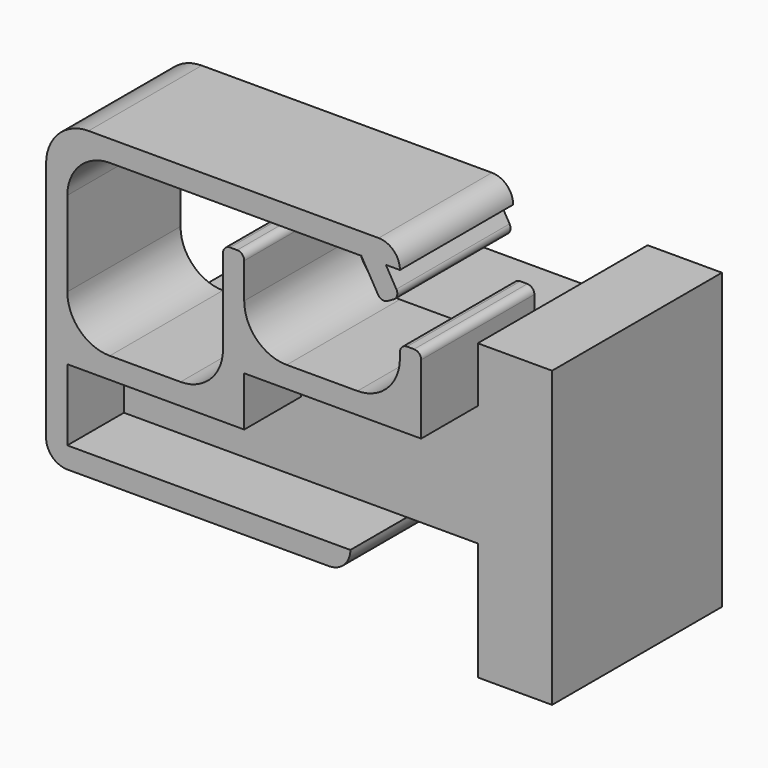
from build123d import *

# Parameters (mm, degrees)
F0_W          = 25
F0_H          = 7
F0_W_2        = 10.5
F0_H_2        = 10.1
F0_H_3        = 16.6735936701
F0_H_4        = 7.8
F1_DEPTH      = 15
F1_DEPTH_BACK = 15
F3_DEPTH      = 10
F3_DEPTH_BACK = 10
F4_R          = 6
F5_R          = 2.99999
F6_R          = 1


# Not quite as in the source:
# - a fillet or chamfer is up to 0.001 mm smaller than in the source, because OpenCascade refuses the exact size


with BuildPart() as f1:
    # F0 (on Front) → F1 (new body, two sides)
    with BuildSketch(Plane.XZ) as f1_sk:
        Polygon((-5.5, 5.1), (-30.5, 5.1), (-30.5, -5), (19.5, -5), (19.5, 5.1), align=None)
        with Locations((7, 8.6)):
            Rectangle(F0_W, F0_H)
        with Locations((24.75, 8.6)):
            Rectangle(F0_W_2, F0_H)
        with Locations((24.75, 0.05)):
            Rectangle(F0_W_2, F0_H_2)
        with Locations((24.75, -13.3367968351)):
            Rectangle(F0_W_2, F0_H_3)
        with Locations((24.75, 16)):
            Rectangle(F0_W_2, F0_H_4)
    extrude(amount=F1_DEPTH)
    extrude(f1_sk.sketch, amount=-F1_DEPTH_BACK)


with BuildPart() as f3:
    # F2 (on face) → F3 (new body, two sides)
    with BuildSketch(Plane.XZ.offset(15)) as f3_sk:
        Polygon((-30.5, -5), (-30.5, 5.1), (-5.5, 5.1), (-5.5, 12.1), (-5.5, 15.1), (-5.5, 27.1), (-8.5, 27.1), (-8.5, 15.1), (-8.5, 8.1), (-30.5, 8.1), (-30.5, 32.1), (11.0402089751, 32.1), (14.5116200045, 32.1), (12.7649962514, 35.1), (1.8319657538, 35.1), (-33.5, 35.1), (-33.5, 8.1), (-33.5, -5), (-33.5, -8), (9.5, -8), (9.5, -5), align=None)
        Polygon((-5.5, 15.1), (-5.5, 12.1), (19.5, 12.1), (19.5, 19.9), (19.5, 22.9), (16.5, 22.9), (16.5, 15.1), align=None)
        Polygon((16.5, 35.1), (12.7649962514, 35.1), (14.5116200045, 32.1), (16.5, 32.1), align=None)
        Polygon((14.5116200045, 32.1), (11.0402089751, 32.1), (13.9073943063, 27.1753240482), (16.5, 28.6847596105), align=None)
    extrude(amount=F3_DEPTH)
    extrude(f3_sk.sketch, amount=-F3_DEPTH_BACK)

    # F4
    f4_edges = [f3.edges().sort_by_distance(p)[0] for p in [
        (-30.5, -15, 8.1),
        (-30.5, -15, 32.1),
        (-8.5, -15, 8.1),
        (16.5, -15, 15.1),
        (-33.5, -15, 35.1),
        (-5.5, -15, 15.1),
    ]]
    fillet(f4_edges, radius=F4_R)

    # F5 (radius 3 in the source; OpenCascade refuses exactly that, so slightly less here)
    f5_edges = [f3.edges().sort_by_distance(p)[0] for p in [
        (-33.5, -15, -8),
        (9.5, -15, -8),
        (16.5, -15, 35.1),
    ]]
    fillet(f5_edges, radius=F5_R)

    # F6
    f6_edges = [f3.edges().sort_by_distance(p)[0] for p in [
        (13.907394, -15, 27.175324),
        (16.5, -15, 28.68476),
        (-8.5, -15, 27.1),
        (-5.5, -15, 27.1),
        (16.5, -15, 22.9),
        (19.5, -15, 22.9),
    ]]
    fillet(f6_edges, radius=F6_R)


solid = Compound([f1.part, f3.part])
